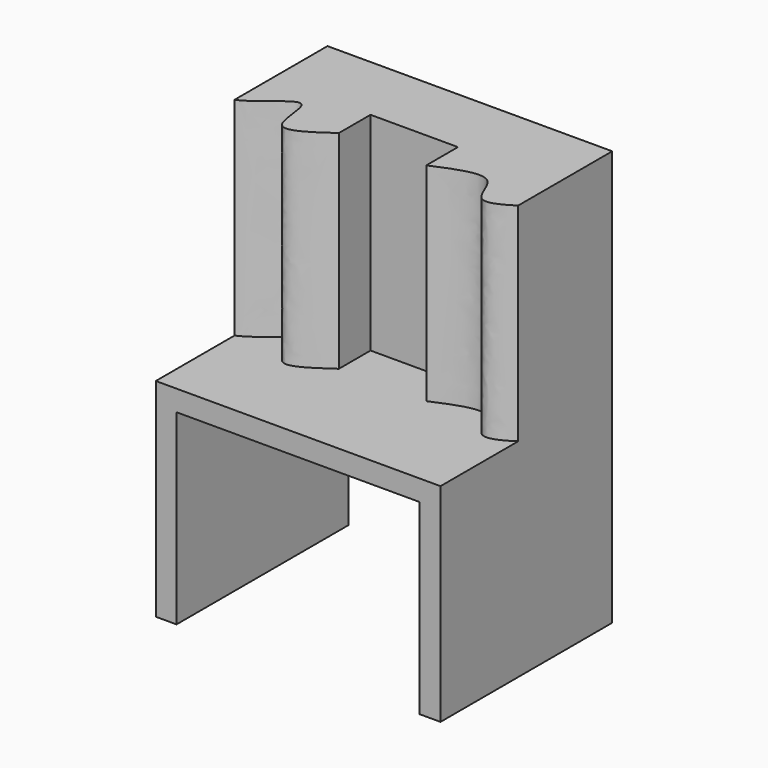
from build123d import *

# Parameters (mm, degrees)
F0_W     = 34.2943547294
F0_H     = 25.8568562567
F1_DEPTH = 25
F2_T     = -2.5
F4_DEPTH = 25


with BuildPart() as f1:
    # F0 (on Top) → F1 (new body)
    with BuildSketch(Plane.XY):
        with Locations((18.5080640949, 12.9284281284)):
            Rectangle(F0_W, F0_H)
    extrude(amount=F1_DEPTH)

    # F2
    f2_openings = [f1.faces().sort_by_distance(p)[0] for p in [
        (18.508064, 25.856856, 12.5),
        (18.508064, 0, 12.5),
        (18.508064, 12.928428, 0),
    ]]
    offset(amount=F2_T, openings=f2_openings)

    # F3 (on face) → F4 (join)
    with BuildSketch(Plane.XY.offset(25)):
        with BuildLine():
            Line((13.2598066702, 17.4573864788), (23.7924046814, 17.4573864788))
            Line((23.7924046814, 17.4573864788), (23.7924046814, 12.689712923))
            add(Edge.make_bspline(
                [(23.7924046814, 12.689712923), (26.3508480961, 13.7881721519), (30.8893318732, 15.7367551698), (31.4069191474, 9.5192493209), (34.1874553016, 10.727986267), (35.6552414596, 11.7030631088)],
                knots=[0, 0, 0, 0, 0.343785498, 0.6098492922, 0.8257809177, 0.8257809177, 0.8257809177, 0.8257809177], degree=3))
            Line((35.6552414596, 11.7030631088), (35.6552414596, 25.8568562567))
            Line((35.6552414596, 25.8568562567), (1.3608867303, 25.8568562567))
            Line((1.3608867303, 25.8568562567), (1.3608867303, 11.8645355105))
            add(Edge.make_bspline(
                [(13.2598066702, 12.689712923), (11.0860272045, 11.1594255192), (6.9288496698, 8.2328745434), (7.8993387733, 18.2466111056), (3.4948427482, 12.7098239865), (1.3608867303, 11.8645355105)],
                knots=[0, 0, 0, 0, 0.2493304721, 0.476824376, 0.7419340081, 0.7419340081, 0.7419340081, 0.7419340081], degree=3))
            Line((13.2598066702, 12.689712923), (13.2598066702, 17.4573864788))
        make_face()
    extrude(amount=F4_DEPTH)


solid = f1.part
